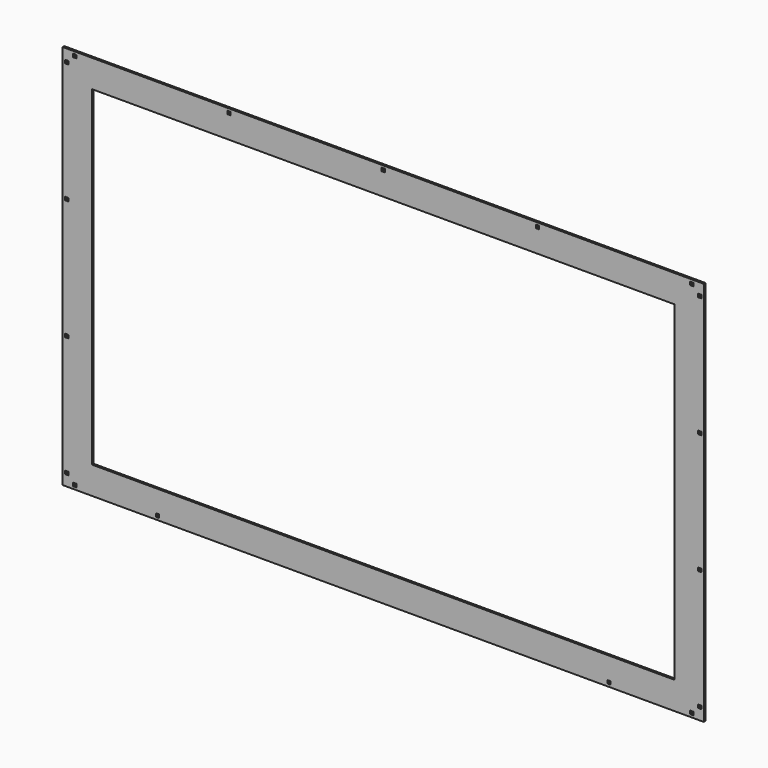
from build123d import *

# Parameters (mm, degrees)
F0_W     = 1016
F0_H     = 611.1875
F0_W_2   = 5.08
F0_H_2   = 5.08
F0_W_3   = 990.6
F0_H_3   = 585.7875
F0_R     = 5.969
F0_W_4   = 951.992
F0_H_4   = 552.45
F0_W_5   = 923.392
F0_H_5   = 523.85
F1_DEPTH = 1.5875


# Not quite as in the source:
# - a feature names something its author has since deleted; it is built from what else it names


with BuildPart() as f1:
    # F0 (on Front) → F1 (new body, symmetric)
    with BuildSketch(Plane.XZ):
        Rectangle(F0_W, F0_H)
        with Locations((-488.95, -299.24375)):
            Rectangle(F0_W_2, F0_H_2, mode=Mode.SUBTRACT)
        Polygon((-504.19, -284.00375), (-501.65, -284.00375), (-499.11, -284.00375), (-499.11, -289.08375), (-504.19, -289.08375), align=None, mode=Mode.SUBTRACT)
        with Locations((-357.84, -299.24375)):
            Rectangle(F0_W_2, F0_H_2, mode=Mode.SUBTRACT)
        Polygon((-504.19, -92.9745833333), (-501.65, -92.9745833333), (-499.11, -92.9745833333), (-499.11, -98.0545833333), (-501.65, -98.0545833333), (-504.19, -98.0545833333), align=None, mode=Mode.SUBTRACT)
        with Locations((357.84, -299.24375)):
            Rectangle(F0_W_2, F0_H_2, mode=Mode.SUBTRACT)
        with Locations((488.95, -299.24375)):
            Rectangle(F0_W_2, F0_H_2, mode=Mode.SUBTRACT)
        with Locations((501.65, -286.54375)):
            Rectangle(F0_W_2, F0_H_2, mode=Mode.SUBTRACT)
        Rectangle(F0_W_3, F0_H_3, mode=Mode.SUBTRACT)
        with Locations((501.65, -95.5145833333)):
            Rectangle(F0_W_2, F0_H_2, mode=Mode.SUBTRACT)
        Polygon((-504.19, 98.0545833333), (-501.65, 98.0545833333), (-499.11, 98.0545833333), (-499.11, 92.9745833333), (-501.65, 92.9745833333), (-504.19, 92.9745833333), align=None, mode=Mode.SUBTRACT)
        Polygon((-501.65, 284.00375), (-504.19, 284.00375), (-504.19, 289.08375), (-499.11, 289.08375), (-499.11, 284.00375), align=None, mode=Mode.SUBTRACT)
        with Locations((-488.95, 299.24375)):
            Circle(F0_R, mode=Mode.SUBTRACT)
        with Locations((-244.475, 299.24375)):
            Rectangle(F0_W_2, F0_H_2, mode=Mode.SUBTRACT)
        with Locations((501.65, 95.5145833333)):
            Rectangle(F0_W_2, F0_H_2, mode=Mode.SUBTRACT)
        with Locations((0, 299.24375)):
            Rectangle(F0_W_2, F0_H_2, mode=Mode.SUBTRACT)
        with Locations((244.475, 299.24375)):
            Rectangle(F0_W_2, F0_H_2, mode=Mode.SUBTRACT)
        with Locations((501.65, 286.54375)):
            Rectangle(F0_W_2, F0_H_2, mode=Mode.SUBTRACT)
        with Locations((488.95, 299.24375)):
            Rectangle(F0_W_2, F0_H_2, mode=Mode.SUBTRACT)
        Rectangle(F0_W_3, F0_H_3)
        Rectangle(F0_W_4, F0_H_4, mode=Mode.SUBTRACT)
        Rectangle(F0_W_4, F0_H_4)
        Rectangle(F0_W_5, F0_H_5, mode=Mode.SUBTRACT)
        with Locations((-488.95, 299.24375)):
            Circle(F0_R)
        with Locations((-488.95, 299.24375)):
            Rectangle(F0_W_2, F0_H_2, mode=Mode.SUBTRACT)
    extrude(amount=F1_DEPTH, both=True)


solid = f1.part
